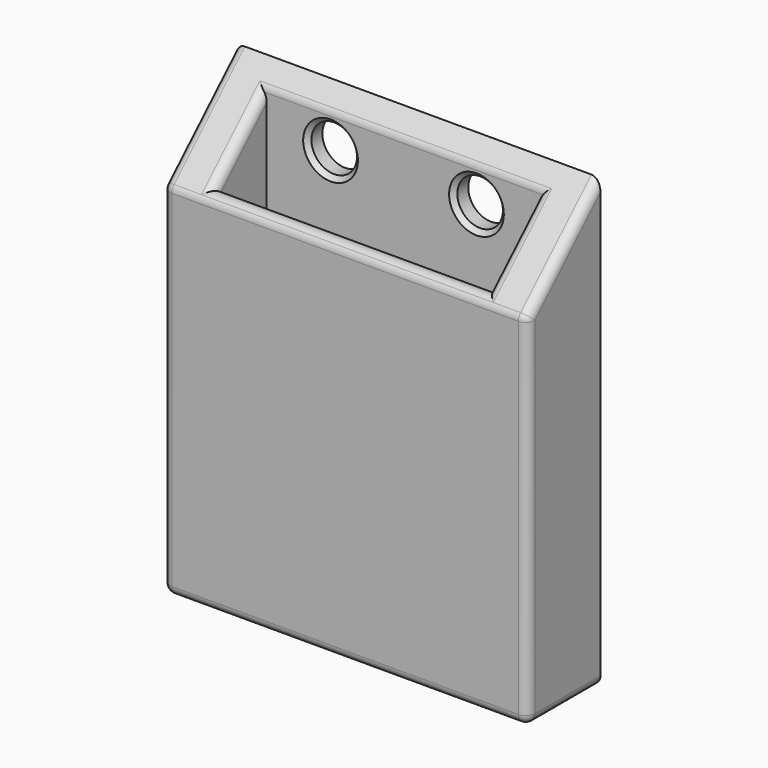
from build123d import *

# Parameters (mm, degrees)
F0_W     = 50.8
F0_H     = 12.7
F0_W_2   = 38.1
F0_H_2   = 7.62
F1_DEPTH = 2.54
F2_DEPTH = 63.5
F4_DEPTH = 50.8
F5_R     = 1.26999
F6_R     = 3.175
F7_DEPTH = 12.7
F8_SIZE  = 0.635


# Not quite as in the source:
# - a fillet or chamfer is up to 0.001 mm smaller than in the source, because OpenCascade refuses the exact size


with BuildPart() as f1:
    # F0 (on Top) → F1 (new body)
    with BuildSketch(Plane.XY):
        Rectangle(F0_W, F0_H)
        Rectangle(F0_W_2, F0_H_2, mode=Mode.SUBTRACT)
        Rectangle(F0_W_2, F0_H_2)
    extrude(amount=-F1_DEPTH)

    # F0 (on Top) → F2 (join)
    with BuildSketch(Plane.XY):
        Rectangle(F0_W, F0_H)
        Rectangle(F0_W_2, F0_H_2, mode=Mode.SUBTRACT)
    extrude(amount=F2_DEPTH)

    # F3 (on Right) → F4 (cut, symmetric)
    with BuildSketch(Plane.YZ):
        Polygon((-17.6573935896, 70.3983381391), (-13.9353135601, 40.1254184544), (17.3301566392, 70.3983381391), align=None)
    extrude(amount=F4_DEPTH, both=True, mode=Mode.SUBTRACT)

    # F5 (radius 1.27 in the source; OpenCascade refuses exactly that, so slightly less here)
    f5_edges = [f1.edges().sort_by_distance(p)[0] for p in [
        (25.4, -6.35, 22.464965),
        (0, -6.35, -2.54),
        (25.4, 0, -2.54),
        (-25.4, 0, -2.54),
        (-25.4, -6.35, 22.464965),
        (0, -6.35, 47.469929),
        (0, -3.81, 49.929295),
        (19.05, 0, 53.618343),
        (0, 3.81, 57.307391),
        (-19.05, 0, 53.618343),
        (-25.4, 0, 53.618343),
        (25.4, 0, 53.618343),
    ]]
    fillet(f5_edges, radius=F5_R)

    # F6 (on Front) → F7 (cut, symmetric)
    with BuildSketch(Plane.XZ):
        with Locations((-10.16, 52.6016924392)):
            Circle(F6_R)
        with Locations((10.16, 52.6016924392)):
            Circle(F6_R)
    extrude(amount=F7_DEPTH, both=True, mode=Mode.SUBTRACT)

    # F8
    f8_edges = [f1.edges().sort_by_distance(p)[0] for p in [
        (-13.335, 3.81, 52.601692),
        (6.985, 3.81, 52.601692),
    ]]
    chamfer(f8_edges, length=F8_SIZE)


solid = f1.part
